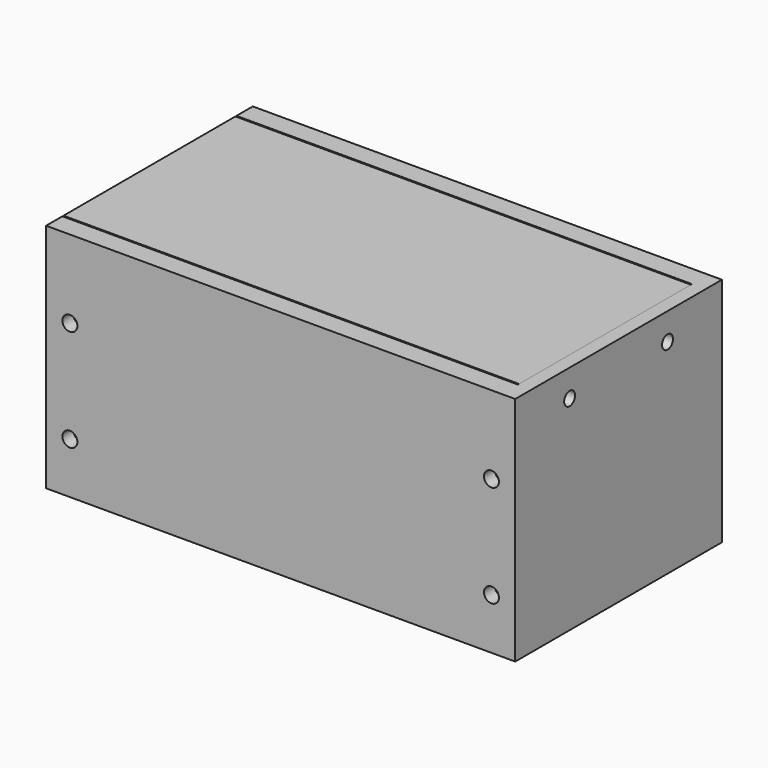
from build123d import *

# Parameters (mm, degrees)
F0_W      = 69
F0_H      = 38
F0_W_2    = 65
F0_H_2    = 34
F1_DEPTH  = 30
F0_W_3    = 62
F0_H_3    = 32
F0_R      = 6.5
F2_DEPTH  = 1.25
F3_START  = 5
F3_DEPTH  = 5
F5_R      = 1.1
F6_DEPTH  = 50
F8_DEPTH  = 69
F9_SIZE   = 0.99999
F10_DEPTH = 67
F11_DEPTH = 4
F12_R     = 1
F13_DEPTH = 69


# Not quite as in the source:
# - a fillet or chamfer is up to 0.001 mm smaller than in the source, because OpenCascade refuses the exact size


with BuildPart() as f1:
    # F0 (on Top) → F1 (new body)
    with BuildSketch(Plane.XY):
        with Locations((22.5, 7.5)):
            Rectangle(F0_W, F0_H)
        with Locations((22.5, 7.5)):
            Rectangle(F0_W_2, F0_H_2, mode=Mode.SUBTRACT)
    extrude(amount=F1_DEPTH)

    # F0 (on Top) → F2 (join)
    with BuildSketch(Plane.XY):
        with Locations((22.5, 7.5)):
            Rectangle(F0_W_2, F0_H_2)
        with Locations((22.5, 7.5)):
            Rectangle(F0_W_3, F0_H_3, mode=Mode.SUBTRACT)
        with Locations((22.5, 7.5)):
            Rectangle(F0_W_3, F0_H_3)
        Circle(F0_R, mode=Mode.SUBTRACT)
        with Locations((15, 0)):
            Circle(F0_R, mode=Mode.SUBTRACT)
        with Locations((30, 0)):
            Circle(F0_R, mode=Mode.SUBTRACT)
        with Locations((45, 0)):
            Circle(F0_R, mode=Mode.SUBTRACT)
        with Locations((0, 15)):
            Circle(F0_R, mode=Mode.SUBTRACT)
        with Locations((15, 15)):
            Circle(F0_R, mode=Mode.SUBTRACT)
        with Locations((30, 15)):
            Circle(F0_R, mode=Mode.SUBTRACT)
        with Locations((45, 15)):
            Circle(F0_R, mode=Mode.SUBTRACT)
        with Locations((0, 15)):
            Circle(F0_R)
        with Locations((15, 15)):
            Circle(F0_R)
        with Locations((30, 15)):
            Circle(F0_R)
        with Locations((45, 15)):
            Circle(F0_R)
        with Locations((45, 0)):
            Circle(F0_R)
        with Locations((15, 0)):
            Circle(F0_R)
        with Locations((30, 0)):
            Circle(F0_R)
        Circle(F0_R)
    extrude(amount=F2_DEPTH)


with BuildPart() as f3:
    # F0 (on Top) → F3 (new body)
    with BuildSketch(Plane.XY.offset(F3_START)):
        with Locations((22.5, 7.5)):
            Rectangle(F0_W_3, F0_H_3)
        Circle(F0_R, mode=Mode.SUBTRACT)
        with Locations((15, 0)):
            Circle(F0_R, mode=Mode.SUBTRACT)
        with Locations((30, 0)):
            Circle(F0_R, mode=Mode.SUBTRACT)
        with Locations((45, 0)):
            Circle(F0_R, mode=Mode.SUBTRACT)
        with Locations((0, 15)):
            Circle(F0_R, mode=Mode.SUBTRACT)
        with Locations((15, 15)):
            Circle(F0_R, mode=Mode.SUBTRACT)
        with Locations((30, 15)):
            Circle(F0_R, mode=Mode.SUBTRACT)
        with Locations((45, 15)):
            Circle(F0_R, mode=Mode.SUBTRACT)
    extrude(amount=F3_DEPTH)


with BuildPart() as f4_1:
    # F4: copy of F3
    add(f3.part.moved(Location((0, 0, 15))))


with BuildPart() as f6_tool:
    # F5 (on face) → F6 (new body, symmetric)
    with BuildSketch(Plane(origin=(0, 26.5, 0), x_dir=(-1, 0, 0), z_dir=(0, 1, 0))):
        with Locations((8.5, 22.5)):
            Circle(F5_R)
        with Locations((8.5, 7.5)):
            Circle(F5_R)
        with Locations((-53.5, 7.5)):
            Circle(F5_R)
        with Locations((-53.5, 22.5)):
            Circle(F5_R)
    extrude(amount=F6_DEPTH, both=True)


with BuildPart() as f1_1:
    add(f1.part)

    # F6: cut by f6_tool
    add(f6_tool.part, mode=Mode.SUBTRACT)

    # F7 (on face) → F8 (join, through all)
    with BuildSketch(Plane(origin=(-12, 0, 0), x_dir=(0, -1, 0), z_dir=(-1, 0, 0))):
        Polygon((-26.5, 34), (-26.5, 30), (-24.5, 30), (-24.5, 32), (-23.5, 32), (-23.5, 34), align=None)
        Polygon((9.5, 30), (11.5, 30), (11.5, 34), (8.5, 34), (8.5, 32), (9.5, 32), align=None)
    extrude(amount=-F8_DEPTH)

    # F9 (size 1 in the source; OpenCascade refuses exactly that, so slightly less here)
    f9_edges = [f1_1.edges().sort_by_distance(p)[0] for p in [
        (22.5, 24.5, 32),
        (22.5, -9.5, 32),
    ]]
    chamfer(f9_edges, length=F9_SIZE)

    # F11 (add, through all): a face of the model
    f11_faces = [f1_1.faces().sort_by_distance(p)[0] for p in [
        (56, 7.5, 30),
    ]]
    extrude(f11_faces, amount=F11_DEPTH)


with BuildPart() as f3_1:
    add(f3.part)

    # F6: cut by f6_tool
    add(f6_tool.part, mode=Mode.SUBTRACT)


with BuildPart() as f4_1_1:
    add(f4_1.part)

    # F6: cut by f6_tool
    add(f6_tool.part, mode=Mode.SUBTRACT)


with BuildPart() as f10:
    # F7 (on face) → F10 (new body, through all)
    with BuildSketch(Plane(origin=(-12, 0, 0), x_dir=(0, -1, 0), z_dir=(-1, 0, 0))):
        Polygon((-24.3, 31.8), (-24.3, 30), (9.3, 30), (9.3, 31.8), (8.3, 31.8), (8.3, 34), (-23.3, 34), (-23.3, 31.8), align=None)
    extrude(amount=-F10_DEPTH)


with BuildPart() as f13_tool:
    # F12 (on face) → F13 (new body, through all)
    with BuildSketch(Plane(origin=(-12, 0, 0), x_dir=(0, -1, 0), z_dir=(-1, 0, 0))):
        with Locations((-16.5, 30)):
            Circle(F12_R)
        with Locations((1.5, 30)):
            Circle(F12_R)
    extrude(amount=-F13_DEPTH)


with BuildPart() as f1_2:
    add(f1_1.part)

    # F13: cut by f13_tool
    add(f13_tool.part, mode=Mode.SUBTRACT)


with BuildPart() as f10_1:
    add(f10.part)

    # F13: cut by f13_tool
    add(f13_tool.part, mode=Mode.SUBTRACT)


solid = Compound([f3_1.part, f4_1_1.part, f1_2.part, f10_1.part])
